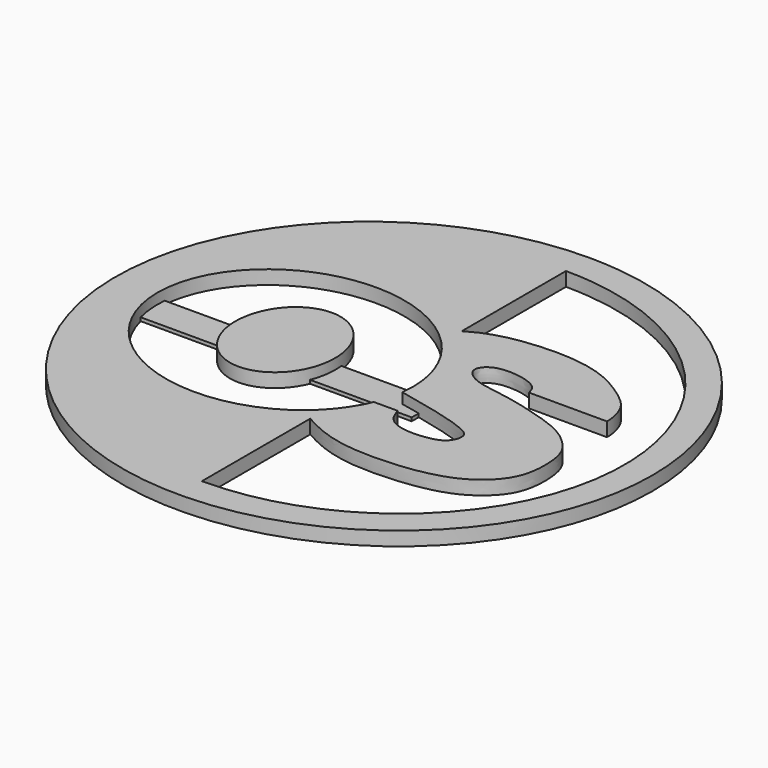
from build123d import *

# Parameters (mm, degrees)
F1_DEPTH = 1
F3_DEPTH = 0.25


with BuildPart() as f1:
    # F0 (on Top) → F1 (new body)
    with BuildSketch(Plane.XY):
        with BuildLine():
            add(Edge.make_bspline(
                [(0, 18.4191223234), (-33.3991670014, 18.4191223234), (-16.6995835007, -9.2095611617), (0, -36.8382446468), (16.6995835007, -9.2095611617), (33.3991670014, 18.4191223234), (0, 18.4191223234)],
                knots=[4.7123889804, 4.7123889804, 4.7123889804, 6.8067840828, 6.8067840828, 8.9011791852, 8.9011791852, 10.9955742876, 10.9955742876, 10.9955742876], degree=2, weights=[1, 0.5, 1, 0.5, 1, 0.5, 1]))
        make_face()
        with BuildLine():
            add(Edge.make_bspline(
                [(2.0296457511, -0.8789825634), (3.5935408506, 11.9068781884), (-10.0880534393, 7.6896991514), (-23.7696477292, 3.4725201143), (-13.6220573579, -5.7034228185), (-3.4744669867, -14.8793657512), (1.5207597149, -2.8075522278)],
                knots=[3.0333950097, 3.0333950097, 3.0333950097, 5.046471668, 5.046471668, 7.0595483262, 7.0595483262, 9.0726249845, 9.0726249845, 9.0726249845], degree=2, weights=[1, 0.534788982, 1, 0.534788982, 1, 0.534788982, 1]))
            add(Edge.make_bspline(
                [(2.0296457511, -0.8789825634), (4.1959245459, -1.3352487154), (7.0386333554, -2.0067184488), (8.1066923125, -2.7397210922), (7.9749546998, -3.4649214618), (7.6692887662, -3.9211820916), (7.1368685251, -4.208759588), (6.078243389, -4.4306087243), (4.5085657916, -4.3898169984), (3.5441273351, -3.7480814881), (3.3371528109, -3.1148922406), (3.2369296532, -2.8075522278)],
                knots=[0, 0, 0, 0, 0.2343670941, 0.335161567, 0.4140464567, 0.4878009759, 0.5638295882, 0.6692431543, 0.7962692486, 0.9012422415, 1, 1, 1, 1], degree=3))
            Line((3.2369296532, -2.8075522278), (1.5207597149, -2.8075522278))
        make_face(mode=Mode.SUBTRACT)
        with BuildLine():
            add(Edge.make_bspline(
                [(0, -16.3369383663), (17.2611761703, -16.3369383663), (17.2611761703, 0), (17.2611761703, 16.3369383663), (0, 16.3369383663)],
                knots=[1.5707963268, 1.5707963268, 1.5707963268, 3.1415926536, 3.1415926536, 4.7123889804, 4.7123889804, 4.7123889804], degree=2, weights=[1, 0.7071067812, 1, 0.7071067812, 1]))
            Line((0, -16.3369383663), (0, -6.6129290499))
            add(Edge.make_bspline(
                [(7.61273643, 3.5189409862), (7.5492835479, 3.731948283), (7.4043802357, 4.2183795026), (6.3786057962, 4.753495834), (4.3933672516, 4.9364243675), (3.4537842591, 4.2023441233), (3.4375255832, 3.4238125679), (4.5750871668, 2.6114661931), (6.8645652894, 2.4165807755), (10.0459375782, 1.5797137112), (11.9738960783, 0.795999988), (13.2030055129, -0.3453323538), (13.8051043581, -1.5032996243), (13.8845839789, -3.8843721599), (13.1328347988, -5.6307377555), (11.3113774877, -7.1214281823), (9.0827977138, -7.7801100525), (6.6845921999, -8.0706595629), (3.7539711861, -8.0518122863), (1.5241242069, -7.4360089256), (0.4813278293, -6.8728627535), (0, -6.6129290499)],
                knots=[0, 0, 0, 0, 0.0321571784, 0.0734353036, 0.1289616072, 0.1692900289, 0.1999726456, 0.2431621905, 0.3037160967, 0.3758908937, 0.4331226424, 0.4823495864, 0.5269622834, 0.5865622852, 0.6407152751, 0.6998339169, 0.7595996736, 0.8211979939, 0.8888719243, 0.9487061553, 1, 1, 1, 1], degree=3))
            Line((7.61273643, 3.5189409862), (13.1968103375, 3.5189409862))
            add(Edge.make_bspline(
                [(0, 6.9871020569), (0.7606964125, 7.4480307471), (2.650742106, 8.2564214656), (8.352208493, 8.5275699755), (11.4734513806, 6.621659875), (12.9392099186, 5.3691184552), (13.2103626649, 4.0083383332), (13.1968103375, 3.5189409862)],
                knots=[0, 0, 0, 0, 0.1967870469, 0.4709237532, 0.6903450292, 0.847859577, 1, 1, 1, 1], degree=3))
            Line((0, 6.9871020569), (0, 16.3369383663))
        make_face(mode=Mode.SUBTRACT)
    extrude(amount=F1_DEPTH)



with BuildPart() as f1b:
    # F0 (on Top) → F1, piece 2 (new body)
    with BuildSketch(Plane.XY):
        with BuildLine():
            add(Edge.make_bspline(
                [(-7.082561031, 4.1916770861), (-13.2823019673, 4.1916770861), (-10.1824314992, -2.095838543), (-7.082561031, -8.3833541721), (-3.9826905628, -2.095838543), (-0.8828200947, 4.1916770861), (-7.082561031, 4.1916770861)],
                knots=[0, 0, 0, 2.0943951024, 2.0943951024, 4.1887902048, 4.1887902048, 6.2831853072, 6.2831853072, 6.2831853072], degree=2, weights=[1, 0.5, 1, 0.5, 1, 0.5, 1]))
        make_face()
    extrude(amount=F1_DEPTH)


with BuildPart() as f1_1:
    add(f1.part)

    add(f1b.part)  # F3 merges F1b
    # F2 (on face) → F3 (join)
    with BuildSketch(Plane(origin=(0, 0, 0), x_dir=(1, 0, 0), z_dir=(0, 0, -1))):
        with BuildLine():
            Line((-10.3085811752, 1.8160907784), (-16.9921703637, 1.8160907784))
            Line((-16.9921703637, 1.8160907784), (-17.0574765652, -0.6002428127))
            Line((-17.0574765652, -0.6002428127), (-10.6250934455, -0.6002428127))
            add(Edge.make_bspline(
                [(-10.6250934455, -0.6002428127), (-10.7813500013, 0.6644204956), (-10.3085811752, 1.8160907784)],
                knots=[1.3959388214, 1.3959388214, 1.3959388214, 2.0050170271, 2.0050170271, 2.0050170271], degree=2, weights=[0.7777261433, 0.8261499779, 0.9591462586]))
        make_face()
        with BuildLine():
            Line((3.4487033263, 1.8160907784), (-3.8565408868, 1.8160907784))
            add(Edge.make_bspline(
                [(-3.8565408868, 1.8160907784), (-3.3837720607, 0.6644204956), (-3.5400286164, -0.6002428127)],
                knots=[4.27816828, 4.27816828, 4.27816828, 4.8872464858, 4.8872464858, 4.8872464858], degree=2, weights=[0.9591462586, 0.8261499779, 0.7777261433]))
            Line((-3.5400286164, -0.6002428127), (3.4487033263, -0.6002428127))
            Line((3.4487033263, -0.6002428127), (3.4487033263, 1.8160907784))
        make_face()
    extrude(amount=-F3_DEPTH)


solid = f1_1.part
